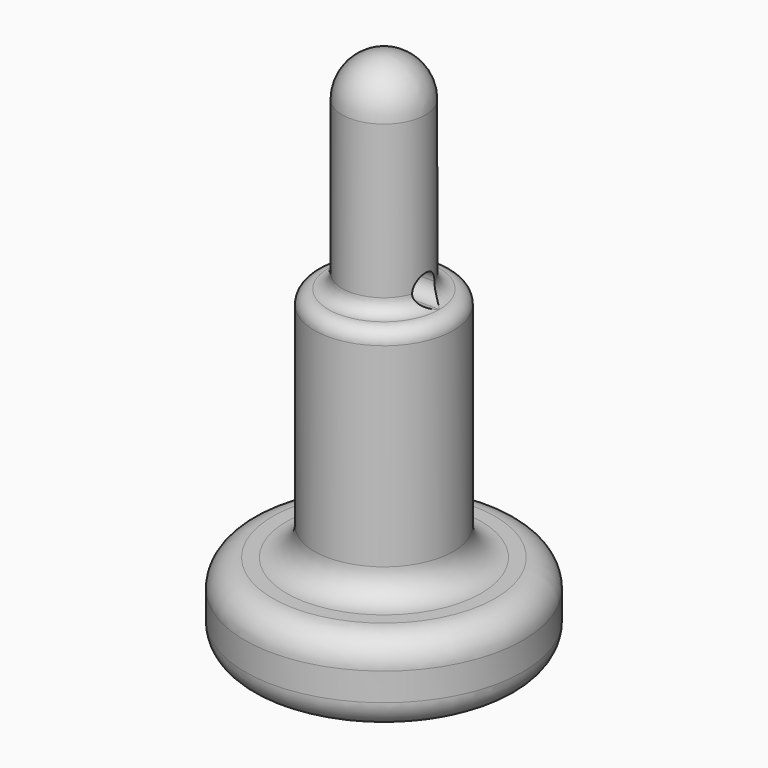
from build123d import *

# Parameters (mm, degrees)
F0_R      = 5
F1_DEPTH  = 3
F2_R      = 2.5
F3_DEPTH  = 8.5
F4_R      = 1.5
F5_DEPTH  = 7.5
F6_R      = 1.5
F7_R      = 1
F8_R      = 0.49999
F10_DEPTH = 2.5


# Not quite as in the source:
# - a fillet or chamfer is up to 0.001 mm smaller than in the source, because OpenCascade refuses the exact size


with BuildPart() as f1:
    # F0 (on Top) → F1 (new body)
    with BuildSketch(Plane.XY):
        Circle(F0_R)
    extrude(amount=F1_DEPTH)

    # F2 (on face) → F3 (join)
    with BuildSketch(Plane.XY.offset(3)):
        Circle(F2_R)
    extrude(amount=F3_DEPTH)

    # F4 (on face) → F5 (join)
    with BuildSketch(Plane.XY.offset(11.5)):
        Circle(F4_R)
    extrude(amount=F5_DEPTH)

    # F6
    f6_edges = [f1.edges().sort_by_distance(p)[0] for p in [
        (-1.5, 0, 19),
    ]]
    fillet(f6_edges, radius=F6_R)

    # F7
    f7_edges = [f1.edges().sort_by_distance(p)[0] for p in [
        (-2.5, 0, 3),
        (-5, 0, 0),
        (-5, 0, 3),
    ]]
    fillet(f7_edges, radius=F7_R)

    # F8 (radius 0.5 in the source; OpenCascade refuses exactly that, so slightly less here)
    f8_edges = [f1.edges().sort_by_distance(p)[0] for p in [
        (-1.5, 0, 11.5),
        (-2.5, 0, 11.5),
    ]]
    fillet(f8_edges, radius=F8_R)

    # F9 (on Right) → F10 (cut, symmetric)
    with BuildSketch(Plane.YZ):
        with BuildLine():
            ThreePointArc((0, 11.5), (0.3535533906, 11.6464466094), (0.5, 12))
            ThreePointArc((0.5, 12), (-0.3535533906, 12.3535533906), (0, 11.5))
        make_face()
    extrude(amount=F10_DEPTH, both=True, mode=Mode.SUBTRACT)


solid = f1.part
